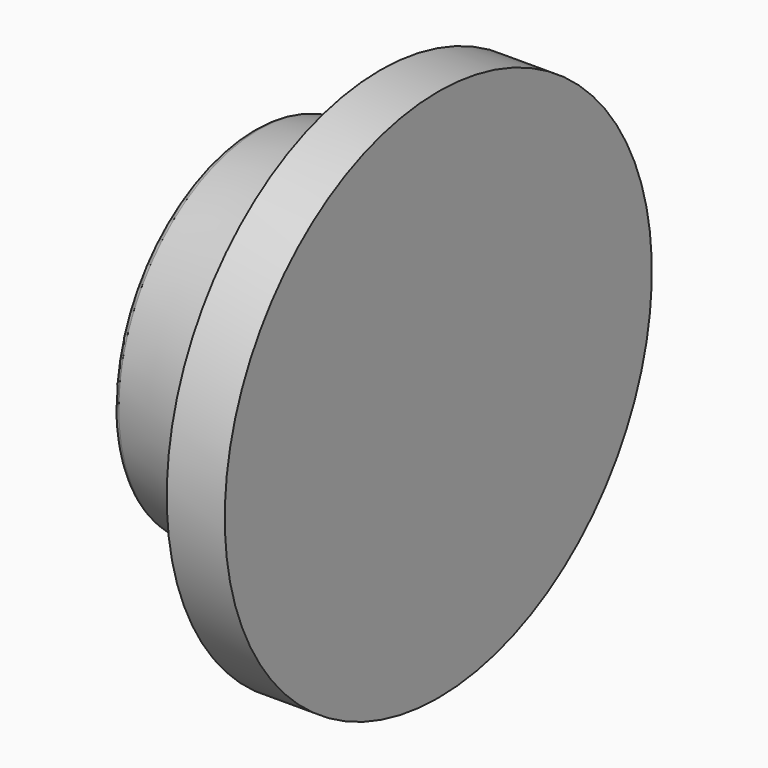
from build123d import *


# Not quite as in the source:
# - a feature of the source that left no trace in its solid (it failed there, or was rolled back) is left out


with BuildPart() as f1:
    # F0 (on Front) → F1 (revolve)
    with BuildSketch(Plane.XZ):
        with BuildLine():
            Line((0, 43.3218007376), (0, 0))
            Line((0, 0), (48, 0))
            Line((48, 0), (48, 69))
            Line((48, 69), (33, 69))
            Line((33, 69), (33, 60))
            Line((33, 60), (30.3564090981, 60))
            ThreePointArc((30.3564090981, 60), (28.9421955357, 59.4142135624), (28.3564090981, 58))
            Line((28.3564090981, 58), (28.3564090981, 50))
            Line((28.3564090981, 50), (1.6527036447, 45.2914162437))
            ThreePointArc((1.6527036447, 45.2914162437), (0.4679111138, 44.607375957), (0, 43.3218007376))
        make_face()
    revolve(axis=Axis((24, 0, 0), (-1, 0, 0)))


solid = f1.part
